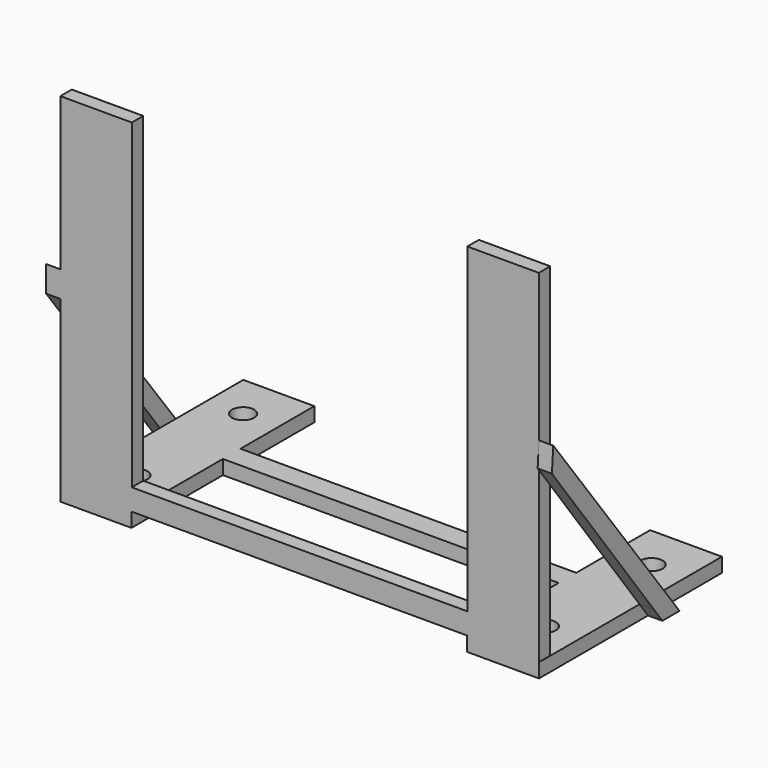
from build123d import *

# Parameters (mm, degrees)
F1_DEPTH = 2
F2_W     = 48.4285755818
F2_H     = 3
F3_DEPTH = 2
F4_R     = 1.55
F4_W     = 9.9543361962
F4_H     = 2
F4_W_2   = 47.0205396414
F4_H_2   = 3.0802486688
F5_DEPTH = 2
F7_DEPTH = 2
F9_DEPTH = 2


# Not quite as in the source:
# - a feature names something its author has since deleted; it is built from what else it names


with BuildPart() as f1:
    # F0 (on Front) → F1 (new body)
    with BuildSketch(Plane.XZ):
        Polygon((-23.5, 24), (-33.5, 24), (-33.5, -24), (-23.5, -24), (-23.5, -21), (-23.5, 20.9024734795), align=None)
    extrude(amount=F1_DEPTH)



with BuildPart() as f1b:
    # F0 (on Front) → F1, piece 2 (new body)
    with BuildSketch(Plane.XZ):
        Polygon((33.5, 24), (23.5, 24), (23.5, 20.9024734795), (23.5, -21), (23.5, -24), (33.5, -24), align=None)
    extrude(amount=F1_DEPTH)


with BuildPart() as f1_1:
    add(f1.part)

    add(f1b.part)  # F3 merges F1b
    # F2 (on Front) → F3 (join)
    with BuildSketch(Plane.XZ):
        with Locations((-0.0266507268, -22.4803313563)):
            Rectangle(F2_W, F2_H)
    extrude(amount=F3_DEPTH)

    # F4 (on face) → F5 (join)
    with BuildSketch(Plane(origin=(0, 0, -24), x_dir=(1, 0, 0), z_dir=(0, 0, -1))):
        Polygon((-23.5456638038, 0), (-33.5, 0), (-33.5, -30.0217941403), (-23.5456638038, -30.0217941403), (-23.5456638038, -17.091145739), (-23.5456638038, -14.0108970702), align=None)
        with Locations((-28.5089425743, -23.7523894757)):
            Circle(F4_R, mode=Mode.SUBTRACT)
        with Locations((-28.5089425743, -5.0747846253)):
            Circle(F4_R, mode=Mode.SUBTRACT)
        with Locations((-28.5228319019, 1)):
            Rectangle(F4_W, F4_H)
        Polygon((33.5320457816, 2), (23.4748758376, 2), (23.4748758376, -2.9849826824), (23.4748758376, -14.0108970702), (23.4748758376, -17.091145739), (23.4748758376, -30.0217941403), (33.5320457816, -30.0217941403), align=None)
        with Locations((28.699381277, -23.7523894757)):
            Circle(F4_R, mode=Mode.SUBTRACT)
        with Locations((28.699381277, -5.0747846253)):
            Circle(F4_R, mode=Mode.SUBTRACT)
        with Locations((-0.0353939831, -15.5510214046)):
            Rectangle(F4_W_2, F4_H_2)
    extrude(amount=F5_DEPTH)

    # F6 (on face) → F7 (join)
    with BuildSketch(Plane.YZ.offset(33.5320457816)):
        Polygon((-2, 3.3605340868), (-2.2395208944, 0), (15.6041713825, -24), (18.5901388697, -24), align=None)
        Polygon((18.5901388697, -24), (15.6041713825, -24), (17.091145739, -26), (20.0952365994, -26), align=None)
    extrude(amount=F7_DEPTH)

    # F8 (on face) → F9 (join)
    with BuildSketch(Plane(origin=(-33.5, 0, 0), x_dir=(0, -1, 0), z_dir=(-1, 0, 0))):
        Polygon((2, 2.6476460043), (0, 0.0077232947), (0, -3.6399227096), (2, -1), align=None)
        Polygon((0, 0.0077232947), (-18.1882016523, -24), (-15.4247525627, -24), (0, -3.6399227096), align=None)
        Polygon((-18.1882016523, -24), (-19.7033975273, -26), (-16.9399484377, -26), (-15.4247525627, -24), align=None)
    extrude(amount=F9_DEPTH)


solid = f1_1.part
